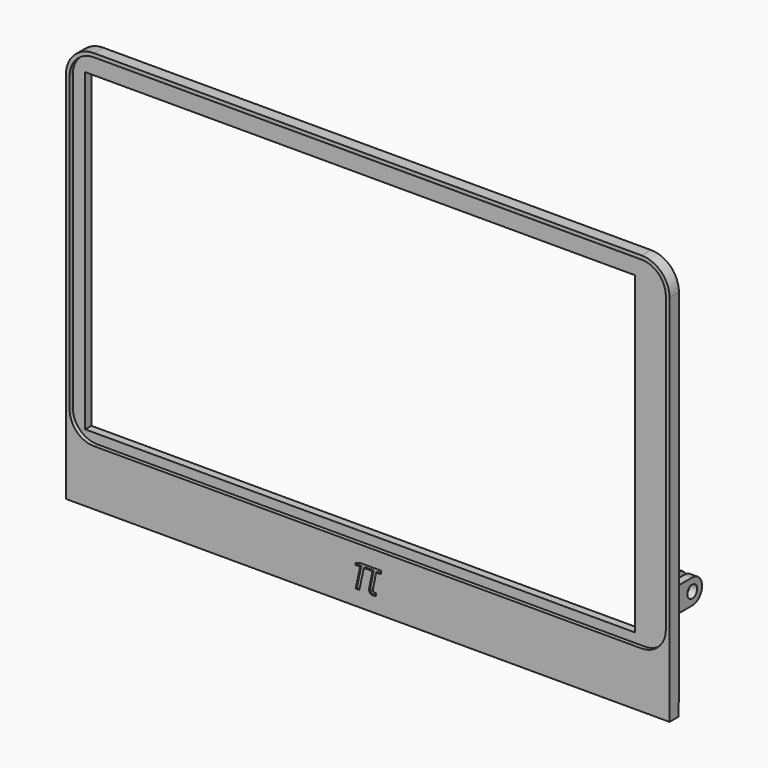
from build123d import *

# Parameters (mm, degrees)
F1_DEPTH  = 3.3
F0_W      = 178
F0_H      = 101.8
F2_DEPTH  = 2.5
F3_W      = 142.8
F3_H      = 4
F4_DEPTH  = 4
F5_R      = 1.99999
F7_D      = 2
F3_W_2    = 26.3
F8_DEPTH  = 0.1
F10_DEPTH = 0.5
F3_W_3    = 2.5
F3_H_2    = 8
F11_DEPTH = 10
F12_R     = 3.99999
F13_R     = 2
F14_DEPTH = 10


# Not quite as in the source:
# - a fillet or chamfer is up to 0.001 mm smaller than in the source, because OpenCascade refuses the exact size


with BuildPart() as f1:
    # F0 (on Front) → F1 (new body)
    with BuildSketch(Plane.XZ):
        with BuildLine():
            ThreePointArc((-75.5207621713, 74.1601898761), (-81.9271496089, 71.5065773137), (-84.5807621713, 65.1001898761))
            Line((-84.5807621713, 65.1001898761), (-84.5807621713, -35.3734344864))
            Line((-84.5807621713, -35.3734344864), (-84.5807621713, -55.8398101239))
            Line((-84.5807621713, -55.8398101239), (110.8192378287, -55.8398101239))
            Line((110.8192378287, -55.8398101239), (110.8192378287, -35.3734344864))
            Line((110.8192378287, -35.3734344864), (110.8192378287, 65.1001898761))
            ThreePointArc((110.8192378287, 65.1001898761), (108.1656252662, 71.5065773137), (101.7592378287, 74.1601898761))
            Line((101.7592378287, 74.1601898761), (-75.5207621713, 74.1601898761))
        make_face()
        with BuildLine():
            ThreePointArc((-83.3807621713, 65.1001898761), (-81.0786214714, 70.6580491763), (-75.5207621713, 72.9601898761))
            Line((-75.5207621713, 72.9601898761), (101.7592378287, 72.9601898761))
            ThreePointArc((101.7592378287, 72.9601898761), (107.3170971288, 70.6580491763), (109.6192378287, 65.1001898761))
            Line((109.6192378287, 65.1001898761), (109.6192378287, -29.9798101239))
            ThreePointArc((109.6192378287, -29.9798101239), (107.3170971288, -35.537669424), (101.7592378287, -37.8398101239))
            Line((101.7592378287, -37.8398101239), (-75.5207621713, -37.8398101239))
            ThreePointArc((-75.5207621713, -37.8398101239), (-81.0786214714, -35.537669424), (-83.3807621713, -29.9798101239))
            Line((-83.3807621713, -29.9798101239), (-83.3807621713, 65.1001898761))
        make_face(mode=Mode.SUBTRACT)
    extrude(amount=F1_DEPTH)

    # F0 (on Front) → F2 (join)
    with BuildSketch(Plane.XZ):
        with BuildLine():
            Line((101.7592378287, 72.9601898761), (-75.5207621713, 72.9601898761))
            ThreePointArc((-75.5207621713, 72.9601898761), (-81.0786214714, 70.6580491763), (-83.3807621713, 65.1001898761))
            Line((-83.3807621713, 65.1001898761), (-83.3807621713, -29.9798101239))
            ThreePointArc((-83.3807621713, -29.9798101239), (-81.0786214714, -35.537669424), (-75.5207621713, -37.8398101239))
            Line((-75.5207621713, -37.8398101239), (101.7592378287, -37.8398101239))
            ThreePointArc((101.7592378287, -37.8398101239), (107.3170971288, -35.537669424), (109.6192378287, -29.9798101239))
            Line((109.6192378287, -29.9798101239), (109.6192378287, 65.1001898761))
            ThreePointArc((109.6192378287, 65.1001898761), (107.3170971288, 70.6580491763), (101.7592378287, 72.9601898761))
        make_face()
        with Locations((9.6192378287, 16.0601898761)):
            Rectangle(F0_W, F0_H, mode=Mode.SUBTRACT)
    extrude(amount=F2_DEPTH)

    # F3 (on face) → F4 (join)
    with BuildSketch(Plane(origin=(0, 0, 0), x_dir=(-1, 0, 0), z_dir=(0, 1, 0))):
        with Locations((-13.1192378287, -53.8398101239)):
            Rectangle(F3_W, F3_H)
    extrude(amount=F4_DEPTH)

    # F5 (radius 2 in the source; OpenCascade refuses exactly that, so slightly less here)
    f5_edges = [f1.edges().sort_by_distance(p)[0] for p in [
        (13.119238, 4, -51.83981),
        (13.119238, 4, -55.83981),
    ]]
    fillet(f5_edges, radius=F5_R)

    # F7 (through all)
    with Locations(Plane.YZ.offset(84.5192378287)):
        with Locations((2, -53.8398101239)):
            Hole(F7_D / 2)

    # F3 (on face) → F8 (cut)
    with BuildSketch(Plane(origin=(0, 0, 0), x_dir=(-1, 0, 0), z_dir=(0, 1, 0))):
        with Locations((-97.6692378287, -53.8398101239)):
            Rectangle(F3_W_2, F3_H)
        with Locations((71.4307621713, -53.8398101239)):
            Rectangle(F3_W_2, F3_H)
    extrude(amount=-F8_DEPTH, mode=Mode.SUBTRACT)

    # F9 (on face) → F10 (join)
    with BuildSketch(Plane.XZ.offset(3.3)):
        with BuildLine():
            Line((101.7592378287, 74.1601898761), (-75.5207621713, 74.1601898761))
            ThreePointArc((-75.5207621713, 74.1601898761), (-81.9271496089, 71.5065773137), (-84.5807621713, 65.1001898761))
            Line((-84.5807621713, 65.1001898761), (-84.5807621713, -55.8398101239))
            Line((-84.5807621713, -55.8398101239), (110.8192378287, -55.8398101239))
            Line((110.8192378287, -55.8398101239), (110.8192378287, 65.1001898761))
            ThreePointArc((110.8192378287, 65.1001898761), (108.1656252662, 71.5065773137), (101.7592378287, 74.1601898761))
        make_face()
        with BuildLine():
            add(Edge.make_bspline(
                [(14.902347951, -49.9172276662), (15.0190761779, -50.0441554468), (15.2457329289, -50.0441554468)],
                knots=[0, 0, 0, 1, 1, 1], degree=2))
            add(Edge.make_bspline(
                [(15.2457329289, -50.0441554468), (15.5585192454, -50.0441554468), (15.8418401843, -49.9308270713)],
                knots=[0, 0, 0, 1, 1, 1], degree=2))
            Line((15.8418401843, -49.9308270713), (15.8418401843, -50.8737191558))
            add(Edge.make_bspline(
                [(15.8418401843, -50.8737191558), (15.3454618994, -51.016512909), (14.8989480998, -51.016512909)],
                knots=[0, 0, 0, 1, 1, 1], degree=2))
            add(Edge.make_bspline(
                [(14.8989480998, -51.016512909), (14.2552429267, -51.016512909), (13.9186576513, -50.6867273361)],
                knots=[0, 0, 0, 1, 1, 1], degree=2))
            add(Edge.make_bspline(
                [(13.9186576513, -50.6867273361), (13.582072376, -50.3569417633), (13.582072376, -49.7835001831)],
                knots=[0, 0, 0, 1, 1, 1], degree=2))
            add(Edge.make_bspline(
                [(13.582072376, -49.7835001831), (13.582072376, -49.3505857885), (13.7090001566, -48.7703445057)],
                knots=[0, 0, 0, 1, 1, 1], degree=2))
            Line((13.7090001566, -48.7703445057), (14.6654916462, -44.144280216))
            Line((14.6654916462, -44.144280216), (11.8662807702, -44.144280216))
            Line((11.8662807702, -44.144280216), (10.4156775633, -50.8737191558))
            Line((10.4156775633, -50.8737191558), (9.212130215, -50.8737191558))
            Line((9.212130215, -50.8737191558), (10.662733422, -44.144280216))
            Line((10.662733422, -44.144280216), (9.0988018395, -44.144280216))
            Line((9.0988018395, -44.144280216), (9.1826648374, -43.6773673088))
            Line((9.1826648374, -43.6773673088), (10.5788704241, -43.1107254311))
            Line((10.5788704241, -43.1107254311), (17.5553652225, -43.1107254311))
            Line((17.5553652225, -43.1107254311), (17.335508174, -44.144280216))
            Line((17.335508174, -44.144280216), (15.8554395894, -44.144280216))
            Line((15.8554395894, -44.144280216), (14.8694827221, -48.8836728813))
            add(Edge.make_bspline(
                [(14.8694827221, -48.8836728813), (14.7856197242, -49.2939216007), (14.7856197242, -49.5840422421)],
                knots=[0, 0, 0, 1, 1, 1], degree=2))
            add(Edge.make_bspline(
                [(14.7856197242, -49.5840422421), (14.7856197242, -49.7902998856), (14.902347951, -49.9172276662)],
                knots=[0, 0, 0, 1, 1, 1], degree=2))
        make_face(mode=Mode.SUBTRACT)
        with BuildLine():
            Line((-83.3807621713, -29.9798101239), (-83.3807621713, 65.1001898761))
            ThreePointArc((-83.3807621713, 65.1001898761), (-81.0786214714, 70.6580491763), (-75.5207621713, 72.9601898761))
            Line((-75.5207621713, 72.9601898761), (101.7592378287, 72.9601898761))
            ThreePointArc((101.7592378287, 72.9601898761), (107.3170971288, 70.6580491763), (109.6192378287, 65.1001898761))
            Line((109.6192378287, 65.1001898761), (109.6192378287, -29.9798101239))
            ThreePointArc((109.6192378287, -29.9798101239), (107.3170971288, -35.537669424), (101.7592378287, -37.8398101239))
            Line((101.7592378287, -37.8398101239), (-75.5207621713, -37.8398101239))
            ThreePointArc((-75.5207621713, -37.8398101239), (-81.0786214714, -35.537669424), (-83.3807621713, -29.9798101239))
        make_face(mode=Mode.SUBTRACT)
    extrude(amount=F10_DEPTH)

    # F3 (on face) → F11 (join)
    with BuildSketch(Plane(origin=(0, 0, 0), x_dir=(-1, 0, 0), z_dir=(0, 1, 0))):
        with Locations((-109.0692378287, -22.8345717341)):
            Rectangle(F3_W_3, F3_H_2)
        with Locations((-104.1692378287, -22.8345717341)):
            Rectangle(F3_W_3, F3_H_2)
    extrude(amount=F11_DEPTH)

    # F12 (radius 4 in the source; OpenCascade refuses exactly that, so slightly less here)
    f12_edges = [f1.edges().sort_by_distance(p)[0] for p in [
        (109.069238, 10, -18.834572),
        (109.069238, 10, -26.834572),
        (104.169238, 10, -18.834572),
        (104.169238, 10, -26.834572),
    ]]
    fillet(f12_edges, radius=F12_R)

    # F13 (on face) → F14 (cut)
    with BuildSketch(Plane.YZ.offset(110.3192378287)):
        with Locations((6, -22.8345717341)):
            Circle(F13_R)
    extrude(amount=-F14_DEPTH, mode=Mode.SUBTRACT)


solid = f1.part
